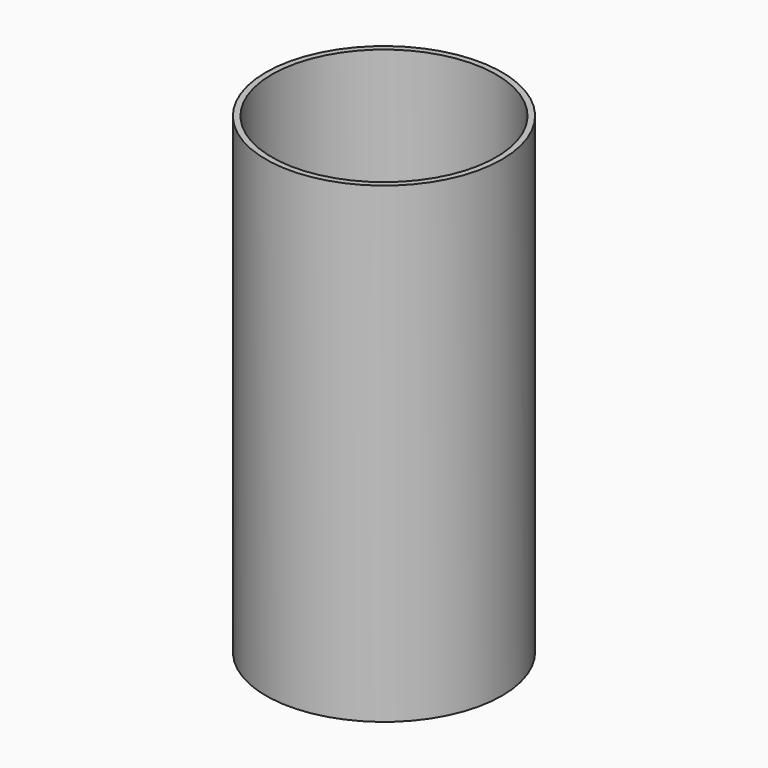
from build123d import *

# Parameters (mm, degrees)
F0_R     = 63.5
F1_DEPTH = 254
F3_D     = 120.65


# Not quite as in the source:
# - a feature names something its author has since deleted; it is built from what else it names


with BuildPart() as f1:
    # F0 (on Top) → F1 (new body)
    with BuildSketch(Plane.XY):
        Circle(F0_R)
    extrude(amount=F1_DEPTH)

    # F3 (through all)
    with Locations(Plane(origin=(0, 0, 0), x_dir=(1, 0, 0), z_dir=(0, 0, -1))):
        with Locations((0, 0)):
            Hole(F3_D / 2)


solid = f1.part
